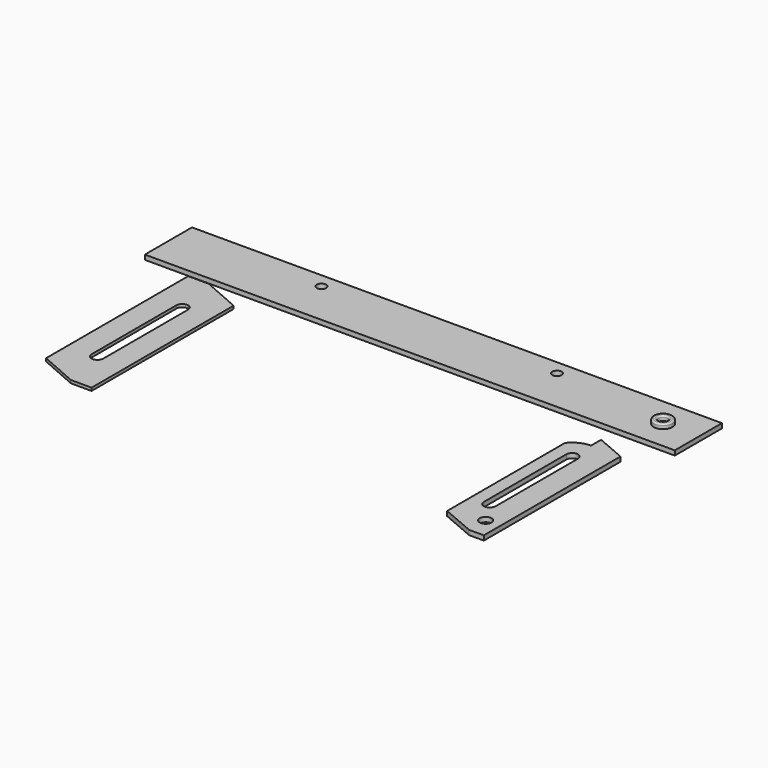
from build123d import *

# Parameters (mm, degrees)
F0_W      = 180
F0_H      = 20
F0_R      = 1.5875
F1_DEPTH  = 1.5875
F2_R      = 2
F3_DEPTH  = 1.5875
F4_R      = 1.5875
F5_DEPTH  = 3.175
F6_R      = 3.175
F6_R_2    = 1.5875
F7_DEPTH  = 1.5875
F6_R_3    = 0.635
F8_DEPTH  = 3.176
F9_R      = 0.508
F10_DEPTH = 1


# Not quite as in the source:
# - a feature names something its author has since deleted; it is built from what else it names


with BuildPart() as f1:
    # F0 (on Top) → F1 (new body)
    with BuildSketch(Plane.XY):
        with Locations((34.1523514688, 29.7559105814)):
            Rectangle(F0_W, F0_H)
        with Locations((112.1523514688, 29.7559105814)):
            Circle(F0_R, mode=Mode.SUBTRACT)
        with Locations((-7.8476485312, 34.7559105814)):
            Circle(F0_R, mode=Mode.SUBTRACT)
        with Locations((72.1523514688, 34.7559105814)):
            Circle(F0_R, mode=Mode.SUBTRACT)
    extrude(amount=F1_DEPTH)


with BuildPart() as f3:
    # F2 (on Top) → F3 (new body)
    with BuildSketch(Plane.XY):
        Polygon((105.1010932944, 12.2813455657), (105.1010932944, 8), (115.1010932944, 8), align=None)
        with BuildLine():
            Line((115.1010932944, 8), (105.1010932944, 8))
            ThreePointArc((105.1010932944, 8), (110.7579475439, 5.6568542495), (113.1010932944, 0))
            ThreePointArc((113.1010932944, 0), (111.4256486147, -4.8989794856), (107.1010932944, -7.7459666924))
            Line((107.1010932944, -7.7459666924), (107.1010932944, -35))
            ThreePointArc((107.1010932944, -35), (105.1010932944, -37), (103.1010932944, -35))
            Line((103.1010932944, -35), (103.1010932944, -7.7459666924))
            ThreePointArc((103.1010932944, -7.7459666924), (100.6847322913, -6.670513885), (98.7510932944, -4.865953144))
            Line((98.7510932944, -4.865953144), (98.7510932944, -43))
            Line((98.7510932944, -43), (110.1010932944, -47.8593272171))
            Line((110.1010932944, -47.8593272171), (115.1010932944, -50))
            Line((115.1010932944, -50), (115.1010932944, 8))
        make_face()
        with Locations((110.1010932944, -43)):
            Circle(F2_R, mode=Mode.SUBTRACT)
        with BuildLine():
            ThreePointArc((113.1010932944, 0), (110.7579475439, 5.6568542495), (105.1010932944, 8))
            ThreePointArc((105.1010932944, 8), (101.5604454124, 7.1738283069), (98.7510932944, 4.865953144))
            Line((98.7510932944, 4.865953144), (98.7510932944, -4.865953144))
            ThreePointArc((98.7510932944, -4.865953144), (100.6847322913, -6.670513885), (103.1010932944, -7.7459666924))
            Line((103.1010932944, -7.7459666924), (103.1010932944, 0))
            ThreePointArc((103.1010932944, 0), (103.686879732, 1.4142135624), (105.1010932944, 2))
            ThreePointArc((105.1010932944, 2), (106.5153068568, 1.4142135624), (107.1010932944, 0))
            Line((107.1010932944, 0), (107.1010932944, -7.7459666924))
            ThreePointArc((107.1010932944, -7.7459666924), (111.4256486147, -4.8989794856), (113.1010932944, 0))
        make_face()
        Polygon((110.1010932944, -50), (115.1010932944, -50), (110.1010932944, -47.8593272171), align=None)
        Polygon((110.1010932944, -47.8593272171), (98.7510932944, -43), (98.7510932944, -45.1406727829), (110.1010932944, -50), align=None)
    extrude(amount=F3_DEPTH)


with BuildPart() as f5:
    # F4 (on face) → F5 (new body)
    with BuildSketch(Plane.XY.offset(1.5875)):
        with Locations((112.1523514688, 29.7559105814)):
            Circle(F4_R)
    extrude(amount=-F5_DEPTH)

    # F6 (on face) → F8 (cut, through all)
    with BuildSketch(Plane.XY.offset(1.5875)):
        with Locations((112.1523514688, 29.7559105814)):
            Circle(F6_R_3)
    extrude(amount=-F8_DEPTH, mode=Mode.SUBTRACT)


with BuildPart() as f7:
    # F6 (on face) → F7 (new body)
    with BuildSketch(Plane.XY.offset(1.5875)):
        with Locations((112.1523514688, 29.7559105814)):
            Circle(F6_R)
        with Locations((112.1523514688, 29.7559105814)):
            Circle(F6_R_2, mode=Mode.SUBTRACT)
    extrude(amount=F7_DEPTH)

    # F9
    f9_edges = [f7.edges().sort_by_distance(p)[0] for p in [
        (110.564851, 29.755911, 3.175),
        (108.977351, 29.755911, 3.175),
    ]]
    fillet(f9_edges, radius=F9_R)


with BuildPart() as f10:
    # F2 (on Top) → F10 (new body)
    with BuildSketch(Plane.XY):
        Polygon((-26.8360394478, -47.8854802153), (-19.8360394478, -47.8854802153), (-19.8360394478, 12.4270197847), (-32.8360394478, 18.1145197847), (-39.8360394478, 18.1145197847), (-39.8360394478, -42.1979802153), align=None)
        with BuildLine():
            Line((-27.8360394478, 3.1145197847), (-27.8360394478, -32.8854802153))
            ThreePointArc((-27.8360394478, -32.8854802153), (-29.8361067273, -34.8854802142), (-31.8360394433, -32.8853456563))
            Line((-31.8360394433, -32.8853456563), (-31.8336240012, 3.0162550804))
            ThreePointArc((-31.8336240012, 3.0162550804), (-31.8360394433, 3.1146543437), (-31.8336107607, 3.2130532811))
            ThreePointArc((-31.8336107607, 3.2130532811), (-29.7867577361, 5.1139125207), (-27.8360394478, 3.1145197847))
        make_face(mode=Mode.SUBTRACT)
    extrude(amount=F10_DEPTH)


solid = Compound([f1.part, f3.part, f5.part, f7.part, f10.part])
